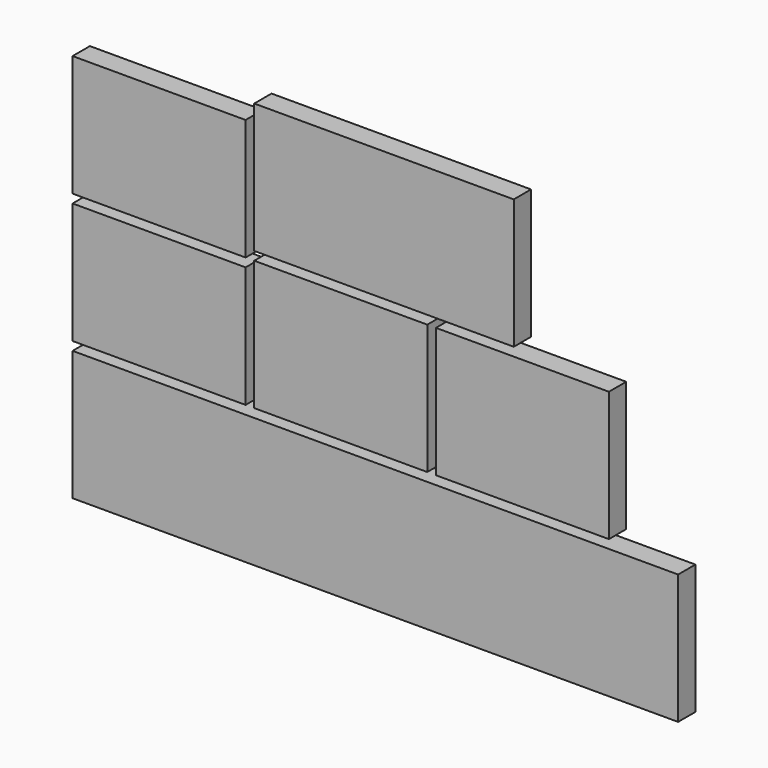
from build123d import *

# Parameters (mm, degrees)
F0_W     = 25.4
F0_H     = 17.78
F1_DEPTH = 3.175
F0_W_2   = 38.1
F0_H_2   = 19.05
F0_W_3   = 88.9


# Not quite as in the source:
# - a length typed as a fraction of an inch, garbled in the dataset ("3 / 203.2 mm" for 3/8 in), is restored


with BuildPart() as f1:
    # F0 (on Front) → F1 (new body)
    with BuildSketch(Plane.XZ):
        with Locations((-44.6465671939, 34.900879418)):
            Rectangle(F0_W, F0_H)
    extrude(amount=F1_DEPTH)


with BuildPart() as f1b:
    # F0 (on Front) → F1, piece 2 (new body)
    with BuildSketch(Plane.XZ):
        with Locations((-11.6265671939, 36.805879418)):
            Rectangle(F0_W_2, F0_H_2)
    extrude(amount=F1_DEPTH)


with BuildPart() as f1c:
    # F0 (on Front) → F1, piece 3 (new body)
    with BuildSketch(Plane.XZ):
        with Locations((-17.9765671939, 16.485879418)):
            Rectangle(F0_W, F0_H_2)
    extrude(amount=F1_DEPTH)


with BuildPart() as f1d:
    # F0 (on Front) → F1, piece 4 (new body)
    with BuildSketch(Plane.XZ):
        with Locations((-44.6465671939, 15.850879418)):
            Rectangle(F0_W, F0_H)
    extrude(amount=F1_DEPTH)


with BuildPart() as f1e:
    # F0 (on Front) → F1, piece 5 (new body)
    with BuildSketch(Plane.XZ):
        with Locations((-12.8965671939, -3.834120582)):
            Rectangle(F0_W_3, F0_H_2)
    extrude(amount=F1_DEPTH)


with BuildPart() as f1f:
    # F0 (on Front) → F1, piece 6 (new body)
    with BuildSketch(Plane.XZ):
        with Locations((8.6934328061, 16.485879418)):
            Rectangle(F0_W, F0_H_2)
    extrude(amount=F1_DEPTH)


solid = Compound([f1.part, f1b.part, f1c.part, f1d.part, f1e.part, f1f.part])
